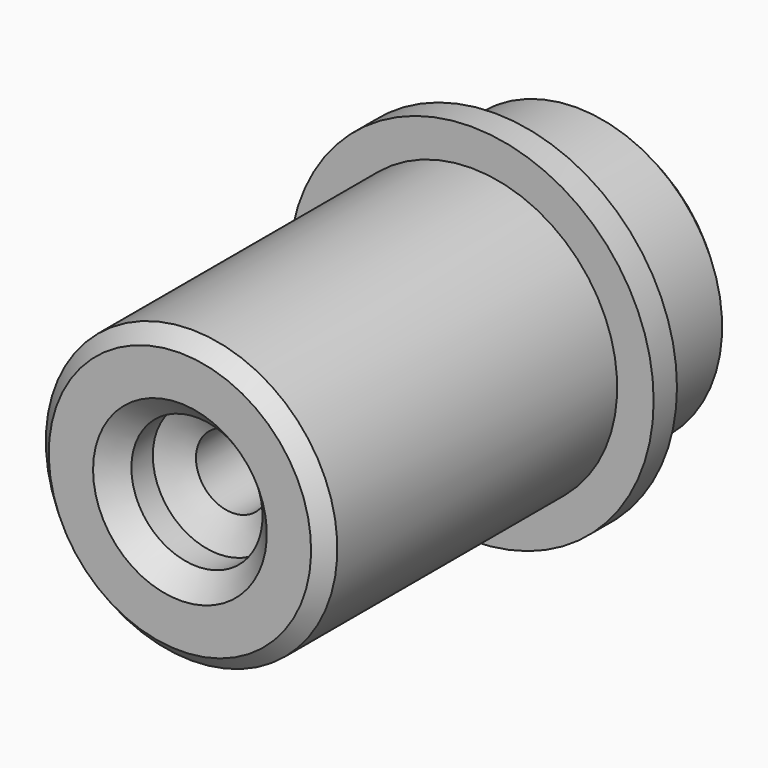
from build123d import *

# Parameters (mm, degrees)
F2_SIZE        = 1
F4_D           = 5
F4_DEPTH       = 15
F4_TIP         = 1.5021515476
F7_D           = 9
F7_DEPTH       = 6.3
F7_CSINK_D     = 17.92
F7_CSINK_ANGLE = 90
F7_TIP         = 2.7038727856


with BuildPart() as f1:
    # F0 (on Right) → F1 (revolve)
    with BuildSketch(Plane.YZ):
        Polygon((-17.5, 10), (-17.5, 0), (17.5, 0), (17.5, 10), (9.5, 10), (9.5, 12.5), (7.5, 12.5), (7.5, 10), align=None)
    revolve(axis=Axis((0, 0, 0), (0, 1, 0)))

    # F2
    f2_edges = [f1.edges().sort_by_distance(p)[0] for p in [
        (0, 17.5, -10),
        (0, -17.5, -10),
    ]]
    chamfer(f2_edges, length=F2_SIZE)

    # F4
    with Locations(Plane.XZ.offset(17.5)):
        with Locations((0, 0)):
            Hole(F4_D / 2, depth=F4_DEPTH)
            with Locations((0, 0, -(F4_DEPTH + F4_TIP / 2))):  # 118° drill point
                Cone(0, F4_D / 2, F4_TIP, mode=Mode.SUBTRACT)

    # F7
    with Locations(Plane.XZ.offset(20.5)):
        with Locations((0, 0)):
            CounterSinkHole(F7_D / 2, F7_CSINK_D / 2, depth=F7_DEPTH, counter_sink_angle=F7_CSINK_ANGLE)
            with Locations((0, 0, -(F7_DEPTH + F7_TIP / 2))):  # 118° drill point
                Cone(0, F7_D / 2, F7_TIP, mode=Mode.SUBTRACT)


solid = f1.part
